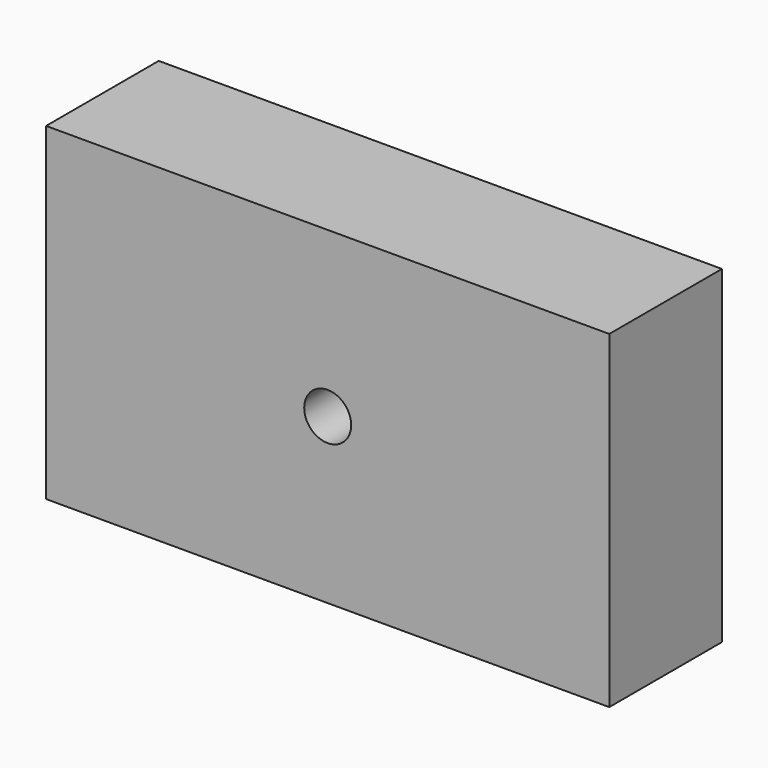
from build123d import *

# Parameters (mm, degrees)
F0_W     = 38.1
F0_H     = 88.9
F1_DEPTH = 152.4
F3_D     = 12.7


# Not quite as in the source:
# - a feature of the source that left no trace in its solid (it failed there, or was rolled back) is left out
# - a length typed as a fraction of an inch, garbled in the dataset ("3 / 203.2 mm" for 3/8 in), is restored


with BuildPart() as f1:
    # F0 (on Right) → F1 (new body)
    with BuildSketch(Plane.YZ):
        Rectangle(F0_W, F0_H)
    extrude(amount=F1_DEPTH)

    # F3 (through all)
    with Locations(Plane.XZ.offset(19.05)):
        with Locations((76.2, 0)):
            Hole(F3_D / 2)


solid = f1.part
